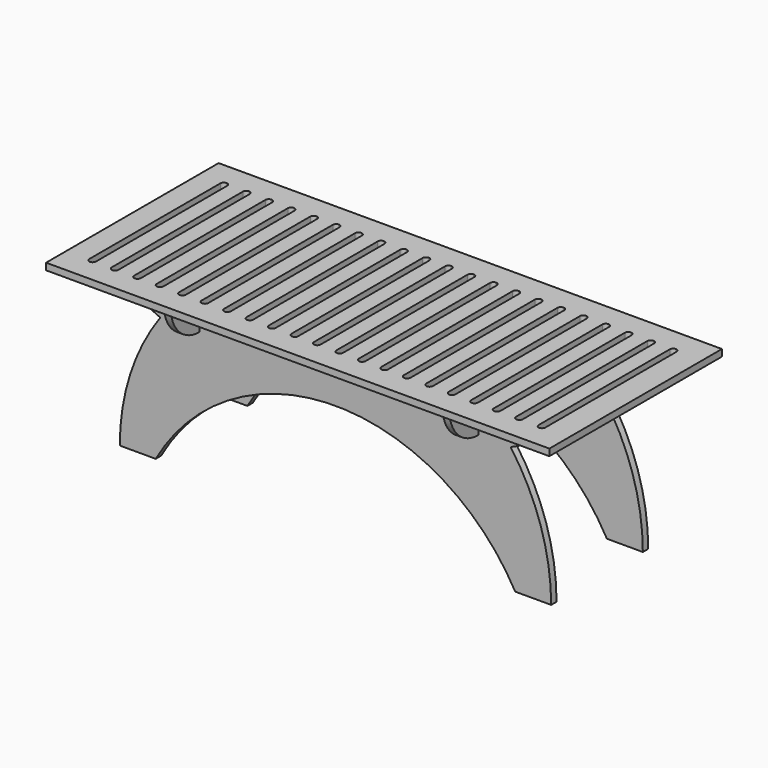
from build123d import *

# Parameters (mm, degrees)
F2_DEPTH  = 19.05
F6_DEPTH  = 19.05
F10_W     = 1422.4
F10_H     = 609.6
F11_DEPTH = 19.05


# Not quite as in the source:
# - a variable given as a bare number and used for a length is read in inches; the dataset says mm whatever the document's units were


with BuildPart() as f2:
    # F1 (on Front) → F2 (new body)
    with BuildSketch(Plane.XZ):
        with BuildLine():
            Line((-99.1726964712, 223.5205044767), (-305.2103381169, 223.5205044767))
            ThreePointArc((-305.2103381169, 223.5205044767), (-256.9834978669, 162.5759153662), (-190.7474908332, 121.9205044767))
            ThreePointArc((-190.7474908332, 121.9205044767), (-275.889481416, -46.8954601989), (-305.2103381169, -233.6794955233))
            Line((-305.2103381169, -233.6794955233), (-203.6103381169, -233.6794955233))
            ThreePointArc((-203.6103381169, -233.6794955233), (304.3896618831, 63.5254637175), (812.3896618831, -233.6794955233))
            Line((812.3896618831, -233.6794955233), (913.9896618831, -233.6794955233))
            ThreePointArc((913.9896618831, -233.6794955233), (884.6688051821, -46.8954601989), (799.5268145994, 121.9205044767))
            ThreePointArc((799.5268145994, 121.9205044767), (865.762821633, 162.5759153662), (913.9896618831, 223.5205044767))
            Line((913.9896618831, 223.5205044767), (707.9520202373, 223.5205044767))
            Line((707.9520202373, 223.5205044767), (707.9520202373, 175.8955044767))
            ThreePointArc((707.9520202373, 175.8955044767), (710.1970842676, 170.4754404464), (704.7770202373, 172.7205044767))
            Line((704.7770202373, 172.7205044767), (692.0770202373, 172.7205044767))
            ThreePointArc((692.0770202373, 172.7205044767), (686.6569562071, 170.4754404464), (688.9020202373, 175.8955044767))
            Line((688.9020202373, 175.8955044767), (688.9020202373, 223.5205044767))
            Line((688.9020202373, 223.5205044767), (-80.1226964712, 223.5205044767))
            Line((-80.1226964712, 223.5205044767), (-80.1226964712, 175.8955044767))
            ThreePointArc((-80.1226964712, 175.8955044767), (-77.8776324409, 170.4754404464), (-83.2976964712, 172.7205044767))
            Line((-83.2976964712, 172.7205044767), (-95.9976964712, 172.7205044767))
            ThreePointArc((-95.9976964712, 172.7205044767), (-101.4177605015, 170.4754404464), (-99.1726964712, 175.8955044767))
            Line((-99.1726964712, 175.8955044767), (-99.1726964712, 223.5205044767))
        make_face()
    extrude(amount=F2_DEPTH)


with BuildPart() as f4_1:
    # F4: instance of F2
    add(f2.part.mirror(Plane(origin=(304.3896618831, -171.45, 60.4125209632), x_dir=(1, 0, 0), z_dir=(0, -1, 0))))


with BuildPart() as f6:
    # F5 (on face) → F6 (new body, through all)
    with BuildSketch(Plane.YZ.offset(-99.1726964712)):
        with BuildLine():
            Line((101.6, 223.5205044767), (-444.5, 223.5205044767))
            ThreePointArc((-444.5, 223.5205044767), (-414.7420489686, 151.6784555081), (-342.9, 121.9205044767))
            Line((-342.9, 121.9205044767), (0, 121.9205044767))
            ThreePointArc((0, 121.9205044767), (71.8420489686, 151.6784555081), (101.6, 223.5205044767))
        make_face()
    extrude(amount=F6_DEPTH)

    # F7: cut F2, F4_1
    add(f2.part, mode=Mode.SUBTRACT)
    add(f4_1.part, mode=Mode.SUBTRACT)


with BuildPart() as f9_1:
    # F9: copy of F6
    add(f6.part.moved(Location((788.0747167085, 0, 0))))


with BuildPart() as f11:
    # F10 (on Top) → F11 (new body)
    with BuildSketch(Plane.XY):
        with Locations((459.0220238209, -197.5034010818)):
            Rectangle(F10_W, F10_H)
        with BuildLine():
            Line((-188.6779761791, -429.2784010818), (-188.6779761791, 34.2715989182))
            ThreePointArc((-188.6779761791, 34.2715989182), (-185.8881682699, 41.006791009), (-179.1529761791, 43.7965989182))
            ThreePointArc((-179.1529761791, 43.7965989182), (-172.4177840883, 41.006791009), (-169.6279761791, 34.2715989182))
            Line((-169.6279761791, 34.2715989182), (-169.6279761791, -429.2784010818))
            ThreePointArc((-169.6279761791, -429.2784010818), (-172.4177840883, -436.0135931726), (-179.1529761791, -438.8034010818))
            ThreePointArc((-179.1529761791, -438.8034010818), (-185.8881682699, -436.0135931726), (-188.6779761791, -429.2784010818))
        make_face(mode=Mode.SUBTRACT)
        with BuildLine():
            ThreePointArc((-125.1779761791, 34.2715989182), (-122.3881682699, 41.006791009), (-115.6529761791, 43.7965989182))
            ThreePointArc((-115.6529761791, 43.7965989182), (-108.9177840883, 41.006791009), (-106.1279761791, 34.2715989182))
            Line((-106.1279761791, 34.2715989182), (-106.1279761791, -429.2784010818))
            ThreePointArc((-106.1279761791, -429.2784010818), (-108.9177840883, -436.0135931726), (-115.6529761791, -438.8034010818))
            ThreePointArc((-115.6529761791, -438.8034010818), (-122.3881682699, -436.0135931726), (-125.1779761791, -429.2784010818))
            Line((-125.1779761791, -429.2784010818), (-125.1779761791, 34.2715989182))
        make_face(mode=Mode.SUBTRACT)
        with BuildLine():
            ThreePointArc((-61.6779761791, 34.2715989182), (-58.8881682699, 41.006791009), (-52.1529761791, 43.7965989182))
            ThreePointArc((-52.1529761791, 43.7965989182), (-45.4177840883, 41.006791009), (-42.6279761791, 34.2715989182))
            Line((-42.6279761791, 34.2715989182), (-42.6279761791, -429.2784010818))
            ThreePointArc((-42.6279761791, -429.2784010818), (-45.4177840883, -436.0135931726), (-52.1529761791, -438.8034010818))
            ThreePointArc((-52.1529761791, -438.8034010818), (-58.8881682699, -436.0135931726), (-61.6779761791, -429.2784010818))
            Line((-61.6779761791, -429.2784010818), (-61.6779761791, 34.2715989182))
        make_face(mode=Mode.SUBTRACT)
        with BuildLine():
            ThreePointArc((1.8220238209, 34.2715989182), (4.6118317301, 41.006791009), (11.3470238209, 43.7965989182))
            ThreePointArc((11.3470238209, 43.7965989182), (18.0822159117, 41.006791009), (20.8720238209, 34.2715989182))
            Line((20.8720238209, 34.2715989182), (20.8720238209, -429.2784010818))
            ThreePointArc((20.8720238209, -429.2784010818), (18.0822159117, -436.0135931726), (11.3470238209, -438.8034010818))
            ThreePointArc((11.3470238209, -438.8034010818), (4.6118317301, -436.0135931726), (1.8220238209, -429.2784010818))
            Line((1.8220238209, -429.2784010818), (1.8220238209, 34.2715989182))
        make_face(mode=Mode.SUBTRACT)
        with BuildLine():
            ThreePointArc((65.3220238209, 34.2715989182), (68.1118317301, 41.006791009), (74.8470238209, 43.7965989182))
            ThreePointArc((74.8470238209, 43.7965989182), (81.5822159117, 41.006791009), (84.3720238209, 34.2715989182))
            Line((84.3720238209, 34.2715989182), (84.3720238209, -429.2784010818))
            ThreePointArc((84.3720238209, -429.2784010818), (81.5822159117, -436.0135931726), (74.8470238209, -438.8034010818))
            ThreePointArc((74.8470238209, -438.8034010818), (68.1118317301, -436.0135931726), (65.3220238209, -429.2784010818))
            Line((65.3220238209, -429.2784010818), (65.3220238209, 34.2715989182))
        make_face(mode=Mode.SUBTRACT)
        with BuildLine():
            ThreePointArc((128.8220238209, 34.2715989182), (131.6118317301, 41.006791009), (138.3470238209, 43.7965989182))
            ThreePointArc((138.3470238209, 43.7965989182), (145.0822159117, 41.006791009), (147.8720238209, 34.2715989182))
            Line((147.8720238209, 34.2715989182), (147.8720238209, -429.2784010818))
            ThreePointArc((147.8720238209, -429.2784010818), (145.0822159117, -436.0135931726), (138.3470238209, -438.8034010818))
            ThreePointArc((138.3470238209, -438.8034010818), (131.6118317301, -436.0135931726), (128.8220238209, -429.2784010818))
            Line((128.8220238209, -429.2784010818), (128.8220238209, 34.2715989182))
        make_face(mode=Mode.SUBTRACT)
        with BuildLine():
            ThreePointArc((192.3220238209, 34.2715989182), (195.1118317301, 41.006791009), (201.8470238209, 43.7965989182))
            ThreePointArc((201.8470238209, 43.7965989182), (208.5822159117, 41.006791009), (211.3720238209, 34.2715989182))
            Line((211.3720238209, 34.2715989182), (211.3720238209, -429.2784010818))
            ThreePointArc((211.3720238209, -429.2784010818), (208.5822159117, -436.0135931726), (201.8470238209, -438.8034010818))
            ThreePointArc((201.8470238209, -438.8034010818), (195.1118317301, -436.0135931726), (192.3220238209, -429.2784010818))
            Line((192.3220238209, -429.2784010818), (192.3220238209, 34.2715989182))
        make_face(mode=Mode.SUBTRACT)
        with BuildLine():
            ThreePointArc((255.8220238209, 34.2715989182), (258.6118317301, 41.006791009), (265.3470238209, 43.7965989182))
            ThreePointArc((265.3470238209, 43.7965989182), (272.0822159117, 41.006791009), (274.8720238209, 34.2715989182))
            Line((274.8720238209, 34.2715989182), (274.8720238209, -429.2784010818))
            ThreePointArc((274.8720238209, -429.2784010818), (272.0822159117, -436.0135931726), (265.3470238209, -438.8034010818))
            ThreePointArc((265.3470238209, -438.8034010818), (258.6118317301, -436.0135931726), (255.8220238209, -429.2784010818))
            Line((255.8220238209, -429.2784010818), (255.8220238209, 34.2715989182))
        make_face(mode=Mode.SUBTRACT)
        with BuildLine():
            ThreePointArc((319.3220238209, 34.2715989182), (322.1118317301, 41.006791009), (328.8470238209, 43.7965989182))
            ThreePointArc((328.8470238209, 43.7965989182), (335.5822159117, 41.006791009), (338.3720238209, 34.2715989182))
            Line((338.3720238209, 34.2715989182), (338.3720238209, -429.2784010818))
            ThreePointArc((338.3720238209, -429.2784010818), (335.5822159117, -436.0135931726), (328.8470238209, -438.8034010818))
            ThreePointArc((328.8470238209, -438.8034010818), (322.1118317301, -436.0135931726), (319.3220238209, -429.2784010818))
            Line((319.3220238209, -429.2784010818), (319.3220238209, 34.2715989182))
        make_face(mode=Mode.SUBTRACT)
        with BuildLine():
            ThreePointArc((382.8220238209, 34.2715989182), (385.6118317301, 41.006791009), (392.3470238209, 43.7965989182))
            ThreePointArc((392.3470238209, 43.7965989182), (399.0822159117, 41.006791009), (401.8720238209, 34.2715989182))
            Line((401.8720238209, 34.2715989182), (401.8720238209, -429.2784010818))
            ThreePointArc((401.8720238209, -429.2784010818), (399.0822159117, -436.0135931726), (392.3470238209, -438.8034010818))
            ThreePointArc((392.3470238209, -438.8034010818), (385.6118317301, -436.0135931726), (382.8220238209, -429.2784010818))
            Line((382.8220238209, -429.2784010818), (382.8220238209, 34.2715989182))
        make_face(mode=Mode.SUBTRACT)
        with BuildLine():
            ThreePointArc((446.3220238209, 34.2715989182), (449.1118317301, 41.006791009), (455.8470238209, 43.7965989182))
            ThreePointArc((455.8470238209, 43.7965989182), (462.5822159117, 41.006791009), (465.3720238209, 34.2715989182))
            Line((465.3720238209, 34.2715989182), (465.3720238209, -429.2784010818))
            ThreePointArc((465.3720238209, -429.2784010818), (462.5822159117, -436.0135931726), (455.8470238209, -438.8034010818))
            ThreePointArc((455.8470238209, -438.8034010818), (449.1118317301, -436.0135931726), (446.3220238209, -429.2784010818))
            Line((446.3220238209, -429.2784010818), (446.3220238209, 34.2715989182))
        make_face(mode=Mode.SUBTRACT)
        with BuildLine():
            ThreePointArc((509.8220238209, 34.2715989182), (512.6118317301, 41.006791009), (519.3470238209, 43.7965989182))
            ThreePointArc((519.3470238209, 43.7965989182), (526.0822159117, 41.006791009), (528.8720238209, 34.2715989182))
            Line((528.8720238209, 34.2715989182), (528.8720238209, -429.2784010818))
            ThreePointArc((528.8720238209, -429.2784010818), (526.0822159117, -436.0135931726), (519.3470238209, -438.8034010818))
            ThreePointArc((519.3470238209, -438.8034010818), (512.6118317301, -436.0135931726), (509.8220238209, -429.2784010818))
            Line((509.8220238209, -429.2784010818), (509.8220238209, 34.2715989182))
        make_face(mode=Mode.SUBTRACT)
        with BuildLine():
            ThreePointArc((573.3220238209, 34.2715989182), (576.1118317301, 41.006791009), (582.8470238209, 43.7965989182))
            ThreePointArc((582.8470238209, 43.7965989182), (589.5822159117, 41.006791009), (592.3720238209, 34.2715989182))
            Line((592.3720238209, 34.2715989182), (592.3720238209, -429.2784010818))
            ThreePointArc((592.3720238209, -429.2784010818), (589.5822159117, -436.0135931726), (582.8470238209, -438.8034010818))
            ThreePointArc((582.8470238209, -438.8034010818), (576.1118317301, -436.0135931726), (573.3220238209, -429.2784010818))
            Line((573.3220238209, -429.2784010818), (573.3220238209, 34.2715989182))
        make_face(mode=Mode.SUBTRACT)
        with BuildLine():
            ThreePointArc((636.8220238209, 34.2715989182), (639.6118317301, 41.006791009), (646.3470238209, 43.7965989182))
            ThreePointArc((646.3470238209, 43.7965989182), (653.0822159117, 41.006791009), (655.8720238209, 34.2715989182))
            Line((655.8720238209, 34.2715989182), (655.8720238209, -429.2784010818))
            ThreePointArc((655.8720238209, -429.2784010818), (653.0822159117, -436.0135931726), (646.3470238209, -438.8034010818))
            ThreePointArc((646.3470238209, -438.8034010818), (639.6118317301, -436.0135931726), (636.8220238209, -429.2784010818))
            Line((636.8220238209, -429.2784010818), (636.8220238209, 34.2715989182))
        make_face(mode=Mode.SUBTRACT)
        with BuildLine():
            ThreePointArc((700.3220238209, 34.2715989182), (703.1118317301, 41.006791009), (709.8470238209, 43.7965989182))
            ThreePointArc((709.8470238209, 43.7965989182), (716.5822159117, 41.006791009), (719.3720238209, 34.2715989182))
            Line((719.3720238209, 34.2715989182), (719.3720238209, -429.2784010818))
            ThreePointArc((719.3720238209, -429.2784010818), (716.5822159117, -436.0135931726), (709.8470238209, -438.8034010818))
            ThreePointArc((709.8470238209, -438.8034010818), (703.1118317301, -436.0135931726), (700.3220238209, -429.2784010818))
            Line((700.3220238209, -429.2784010818), (700.3220238209, 34.2715989182))
        make_face(mode=Mode.SUBTRACT)
        with BuildLine():
            ThreePointArc((763.8220238209, 34.2715989182), (766.6118317301, 41.006791009), (773.3470238209, 43.7965989182))
            ThreePointArc((773.3470238209, 43.7965989182), (780.0822159117, 41.006791009), (782.8720238209, 34.2715989182))
            Line((782.8720238209, 34.2715989182), (782.8720238209, -429.2784010818))
            ThreePointArc((782.8720238209, -429.2784010818), (780.0822159117, -436.0135931726), (773.3470238209, -438.8034010818))
            ThreePointArc((773.3470238209, -438.8034010818), (766.6118317301, -436.0135931726), (763.8220238209, -429.2784010818))
            Line((763.8220238209, -429.2784010818), (763.8220238209, 34.2715989182))
        make_face(mode=Mode.SUBTRACT)
        with BuildLine():
            ThreePointArc((827.3220238209, 34.2715989182), (830.1118317301, 41.006791009), (836.8470238209, 43.7965989182))
            ThreePointArc((836.8470238209, 43.7965989182), (843.5822159117, 41.006791009), (846.3720238209, 34.2715989182))
            Line((846.3720238209, 34.2715989182), (846.3720238209, -429.2784010818))
            ThreePointArc((846.3720238209, -429.2784010818), (843.5822159117, -436.0135931726), (836.8470238209, -438.8034010818))
            ThreePointArc((836.8470238209, -438.8034010818), (830.1118317301, -436.0135931726), (827.3220238209, -429.2784010818))
            Line((827.3220238209, -429.2784010818), (827.3220238209, 34.2715989182))
        make_face(mode=Mode.SUBTRACT)
        with BuildLine():
            ThreePointArc((890.8220238209, 34.2715989182), (893.6118317301, 41.006791009), (900.3470238209, 43.7965989182))
            ThreePointArc((900.3470238209, 43.7965989182), (907.0822159117, 41.006791009), (909.8720238209, 34.2715989182))
            Line((909.8720238209, 34.2715989182), (909.8720238209, -429.2784010818))
            ThreePointArc((909.8720238209, -429.2784010818), (907.0822159117, -436.0135931726), (900.3470238209, -438.8034010818))
            ThreePointArc((900.3470238209, -438.8034010818), (893.6118317301, -436.0135931726), (890.8220238209, -429.2784010818))
            Line((890.8220238209, -429.2784010818), (890.8220238209, 34.2715989182))
        make_face(mode=Mode.SUBTRACT)
        with BuildLine():
            ThreePointArc((954.3220238209, 34.2715989182), (957.1118317301, 41.006791009), (963.8470238209, 43.7965989182))
            ThreePointArc((963.8470238209, 43.7965989182), (970.5822159117, 41.006791009), (973.3720238209, 34.2715989182))
            Line((973.3720238209, 34.2715989182), (973.3720238209, -429.2784010818))
            ThreePointArc((973.3720238209, -429.2784010818), (970.5822159117, -436.0135931726), (963.8470238209, -438.8034010818))
            ThreePointArc((963.8470238209, -438.8034010818), (957.1118317301, -436.0135931726), (954.3220238209, -429.2784010818))
            Line((954.3220238209, -429.2784010818), (954.3220238209, 34.2715989182))
        make_face(mode=Mode.SUBTRACT)
        with BuildLine():
            ThreePointArc((1017.8220238209, 34.2715989182), (1020.6118317301, 41.006791009), (1027.3470238209, 43.7965989182))
            ThreePointArc((1027.3470238209, 43.7965989182), (1034.0822159117, 41.006791009), (1036.8720238209, 34.2715989182))
            Line((1036.8720238209, 34.2715989182), (1036.8720238209, -429.2784010818))
            ThreePointArc((1036.8720238209, -429.2784010818), (1034.0822159117, -436.0135931726), (1027.3470238209, -438.8034010818))
            ThreePointArc((1027.3470238209, -438.8034010818), (1020.6118317301, -436.0135931726), (1017.8220238209, -429.2784010818))
            Line((1017.8220238209, -429.2784010818), (1017.8220238209, 34.2715989182))
        make_face(mode=Mode.SUBTRACT)
        with BuildLine():
            ThreePointArc((1081.3220238209, 34.2715989182), (1084.1118317301, 41.006791009), (1090.8470238209, 43.7965989182))
            ThreePointArc((1090.8470238209, 43.7965989182), (1097.5822159117, 41.006791009), (1100.3720238209, 34.2715989182))
            Line((1100.3720238209, 34.2715989182), (1100.3720238209, -429.2784010818))
            ThreePointArc((1100.3720238209, -429.2784010818), (1097.5822159117, -436.0135931726), (1090.8470238209, -438.8034010818))
            ThreePointArc((1090.8470238209, -438.8034010818), (1084.1118317301, -436.0135931726), (1081.3220238209, -429.2784010818))
            Line((1081.3220238209, -429.2784010818), (1081.3220238209, 34.2715989182))
        make_face(mode=Mode.SUBTRACT)
    extrude(amount=F11_DEPTH)


with BuildPart() as f11_1:
    # F13: moved
    add(f11.part.moved(Location((-154.6323619378, 26.0534010818, 223.5205044767))))


solid = Compound([f2.part, f4_1.part, f6.part, f9_1.part, f11_1.part])
